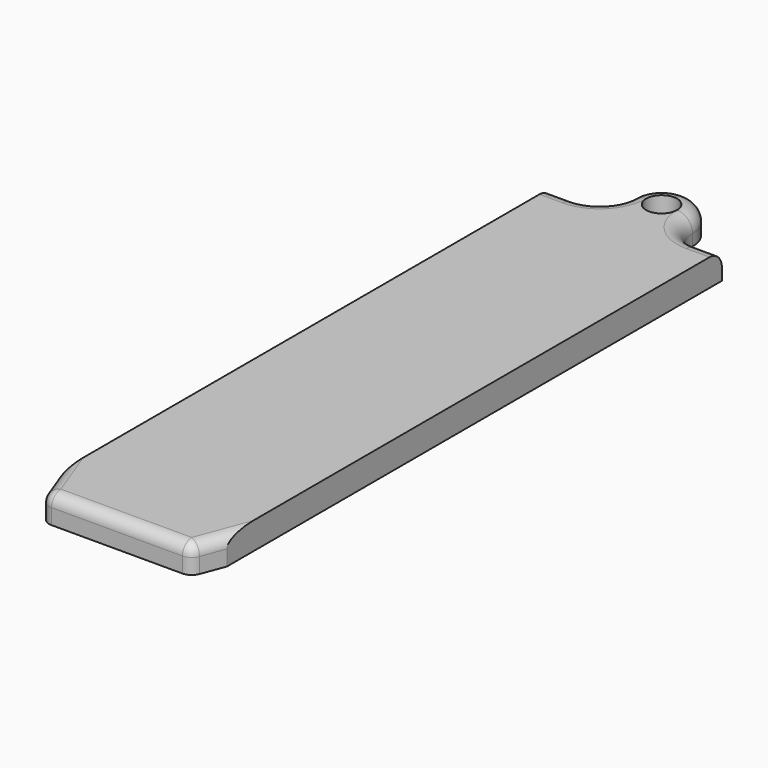
from build123d import *

# Parameters (mm, degrees)
F0_R     = 1
F1_DEPTH = 1.75
F2_R     = 0.99999
F4_DEPTH = 25
F5_R     = 0.75


# Not quite as in the source:
# - a fillet or chamfer is up to 0.001 mm smaller than in the source, because OpenCascade refuses the exact size


with BuildPart() as f1:
    # F0 (on Top) → F1 (new body)
    with BuildSketch(Plane.XY):
        with BuildLine():
            Line((-5.5, -21), (5.5, -21))
            Line((5.5, -21), (5.5, 21))
            Line((5.5, 21), (4, 21))
            ThreePointArc((4, 21), (2.5857864376, 21.5857864376), (2, 23))
            ThreePointArc((2, 23), (1.4142135624, 24.4142135624), (0, 25))
            ThreePointArc((0, 25), (-1.4142135624, 24.4142135624), (-2, 23))
            ThreePointArc((-2, 23), (-2.5857864376, 21.5857864376), (-4, 21))
            Line((-4, 21), (-5.5, 21))
            Line((-5.5, 21), (-5.5, -21))
        make_face()
        with Locations((0, 23)):
            Circle(F0_R, mode=Mode.SUBTRACT)
    extrude(amount=F1_DEPTH)

    # F2 (radius 1 in the source; OpenCascade refuses exactly that, so slightly less here)
    f2_edges = [f1.edges().sort_by_distance(p)[0] for p in [
        (-2.585786, 21.585786, 1.75),
    ]]
    fillet(f2_edges, radius=F2_R)

    # F3 (on face) → F4 (cut)
    with BuildSketch(Plane.XY.offset(1.75)):
        Polygon((-5.5, -21), (-4.75, -21), (-5.5, -19), align=None)
        Polygon((5.5, -19), (4.75, -21), (5.5, -21), align=None)
    extrude(amount=-F4_DEPTH, mode=Mode.SUBTRACT)

    # F5
    f5_edges = [f1.edges().sort_by_distance(p)[0] for p in [
        (-5.125, -20, 1.75),
        (0, -21, 1.75),
        (5.125, -20, 1.75),
        (-4.75, -21, 0.875),
        (4.75, -21, 0.875),
    ]]
    fillet(f5_edges, radius=F5_R)


solid = f1.part
